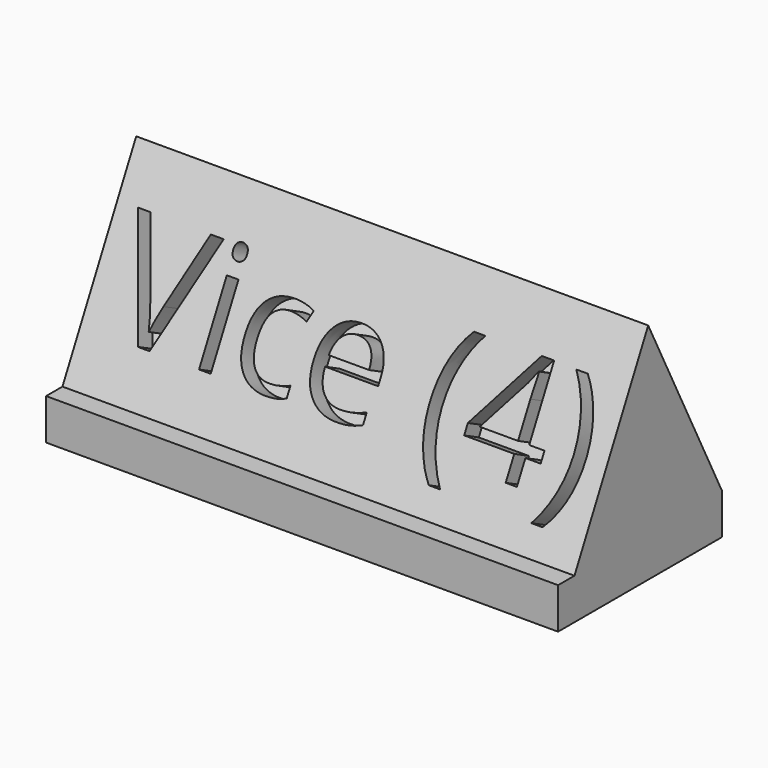
from build123d import *

# Parameters (mm, degrees)
F1_DEPTH     = 63.5
F2_TEXT_SIZE = 17.8722753346
F3_DEPTH     = 2.54


# Not quite as in the source:
# - Text() gives the source's letters only with a copy of the font that has no kerning and outlines rounded to 1/6400 em; it was checked with that copy


with BuildPart() as f1:
    # F0 (on Right) → F1 (new body)
    with BuildSketch(Plane.YZ):
        Polygon((0, 5.08), (0, 0), (25.4, 0), (25.4, 5.08), (13.97, 27.7629252964), (2.54, 5.08), align=None)
    extrude(amount=F1_DEPTH)

    # F2 (on face) → F3 (cut)
    with BuildSketch(Plane(origin=(0, -0.0158132767, 0.0079683617), x_dir=(1, 0, 0), z_dir=(0, -0.893028555, 0.45))):
        with Locations((2.54, 11.8615468184)):
            Text('Vice (4)', F2_TEXT_SIZE, font='Open Sans', text_align=(TextAlign.LEFT, TextAlign.BOTTOM))
    extrude(amount=-F3_DEPTH, mode=Mode.SUBTRACT)


solid = f1.part
